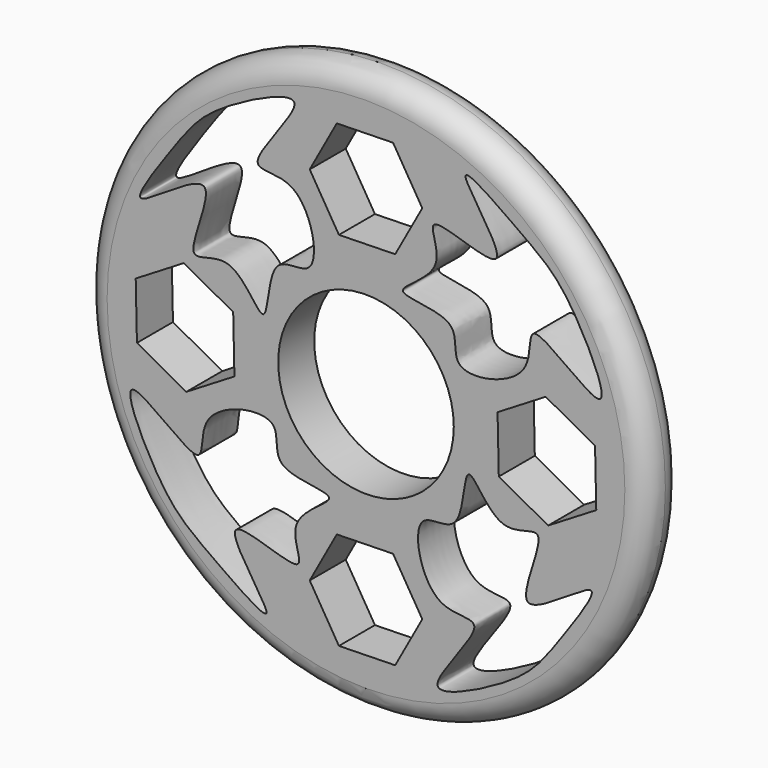
from build123d import *

# Parameters (mm, degrees)
F0_R            = 31.75
F0_R_2          = 9.906
F1_DEPTH        = 5.08
F3_DEPTH        = 25.4
F3_COPIES_COUNT = 4
F5_DEPTH        = 25.4
F5_COPIES_COUNT = 4
F6_R            = 2.53999


# Not quite as in the source:
# - a fillet or chamfer is up to 0.001 mm smaller than in the source, because OpenCascade refuses the exact size
# - a pattern or mirror of a feature is missing from the dataset's text; its kind, count and spacing are read off the source's solid


with BuildPart() as f1:
    # F0 (on Front) → F1 (new body)
    with BuildSketch(Plane.XZ):
        Circle(F0_R)
        Circle(F0_R_2, mode=Mode.SUBTRACT)
    extrude(amount=F1_DEPTH)

    # F2 (on face) → F3 (cut)
    with BuildSketch(Plane.XZ.offset(5.08)):
        Polygon((3.295605247, 14.9843848394), (6.35, 20.5532776252), (3.054394753, 25.9829074674), (-3.295605247, 25.8436445238), (-6.35, 20.274751738), (-3.054394753, 14.8451218958), align=None)
    f3 = extrude(amount=-F3_DEPTH, mode=Mode.SUBTRACT)

    # F3_copies: F3 ×4 about axis
    f3_copies_axis = Axis((0, 0, 0), (0, 1, 0))
    for i in range(1, F3_COPIES_COUNT):
        add(f3.rotate(f3_copies_axis, i * 360 / F3_COPIES_COUNT), mode=Mode.SUBTRACT)

    # F4 (on face) → F5 (cut)
    with BuildSketch(Plane.XZ.offset(5.08)):
        with BuildLine():
            add(Edge.make_bspline(
                [(-25.2823196352, 11.2266652286), (-26.2167473391, 11.1719195171), (-20.851844375, 18.638002536), (-17.9735815327, 22.8236193788), (-3.4488533652, 29.761678005), (-15.3695380337, 17.1898336012), (-6.8911828605, 19.7725553025), (-4.5327384136, 8.6157936045), (-11.2917188218, 11.4208853363), (-10.7900429942, 0.622794269), (-14.8411551523, 10.0301172445), (-21.7400964963, 5.1099364781), (-14.6224946962, 19.3767771256), (-24.2842285899, 11.2851408112), (-25.2823196352, 11.2266652286)],
                knots=[0, 0, 0, 0, 0.0869034867, 0.1833368975, 0.2803321465, 0.3758280265, 0.4430572841, 0.5338443119, 0.5987211427, 0.6767905103, 0.7539012784, 0.8193857357, 0.9071757061, 1, 1, 1, 1], degree=3))
        make_face()
    f5 = extrude(amount=-F5_DEPTH, mode=Mode.SUBTRACT)

    # F5_copies: F5 ×4 about axis
    f5_copies_axis = Axis((0, 0, 0), (0, 1, 0))
    for i in range(1, F5_COPIES_COUNT):
        add(f5.rotate(f5_copies_axis, i * 360 / F5_COPIES_COUNT), mode=Mode.SUBTRACT)

    # F6 (radius 2.54 in the source; OpenCascade refuses exactly that, so slightly less here)
    f6_edges = [f1.edges().sort_by_distance(p)[0] for p in [
        (-31.75, 0, 0),
        (-31.75, -5.08, 0),
    ]]
    fillet(f6_edges, radius=F6_R)


solid = f1.part
